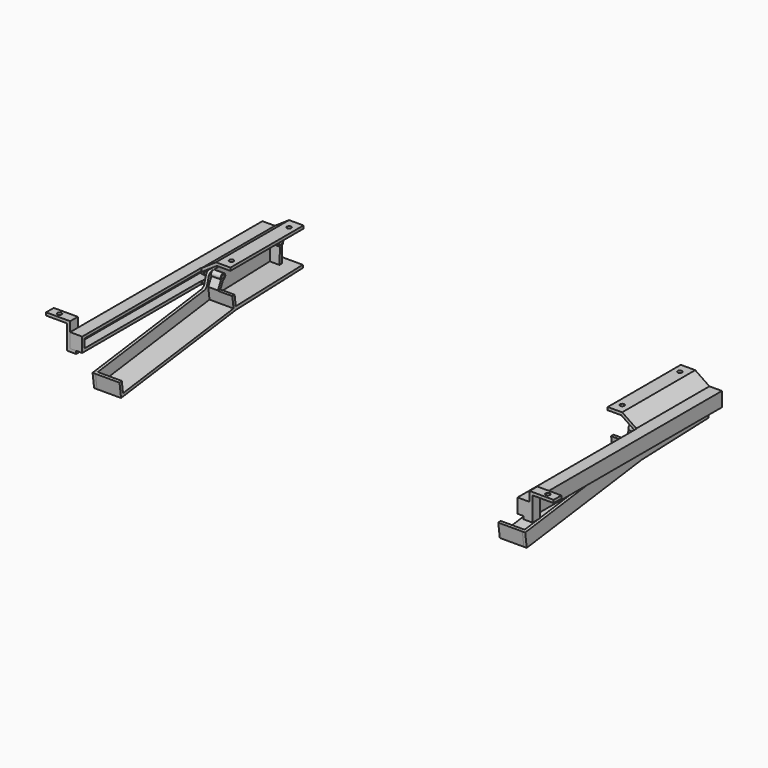
from build123d import *
from build123d import SkipClean  # not in build123d's __all__

# Parameters (mm, degrees)
F0_R      = 4
F0_R_2    = 1.5
F1_DEPTH  = 1.5
F4_DEPTH  = 3
F5_W      = 250
F5_H      = 3
F6_DEPTH  = 10
F8_DEPTH  = 10
F11_DEPTH = 3
F12_R     = 1.75
F13_DEPTH = 3
F15_DEPTH = 25
F19_DEPTH = 10
F24_DEPTH = 3
F27_DEPTH = 250
F28_R     = 2.25
F29_DEPTH = 3
F30_W     = 15.1967487764
F30_H     = 155
F31_DEPTH = 25.001
F36_DEPTH = 3
F37_R     = 5
F40_DEPTH = 10
F41_R     = 2.25
F42_DEPTH = 3


# Not quite as in the source:
# - after a boolean that leaves OpenCascade's solid faulty, fix() repairs it


with BuildPart() as f1:
    # F0 (on Right) → F1 (new body, symmetric)
    with BuildSketch(Plane.YZ):
        Circle(F0_R)
        Circle(F0_R_2, mode=Mode.SUBTRACT)
    extrude(amount=F1_DEPTH, both=True)


with BuildPart() as f1b:
    # F0 (on Right) → F1, piece 2 (new body, symmetric)
    with BuildSketch(Plane.YZ):
        with Locations((75, 0)):
            Circle(F0_R)
        with Locations((75, 0)):
            Circle(F0_R_2, mode=Mode.SUBTRACT)
    extrude(amount=F1_DEPTH, both=True)


with BuildPart() as f4:
    # F3 (on offset) → F4 (new body)
    with BuildSketch(Plane.YZ.offset(-9)):
        Polygon((85, -7.5), (85, 0), (85, 7.5), (-165, 7.5), (-165, -7.5), align=None)
    extrude(amount=F4_DEPTH)

    # F5 (on face) → F6 (join)
    with BuildSketch(Plane.YZ.offset(-6)):
        with Locations((-40, 6)):
            Rectangle(F5_W, F5_H)
    extrude(amount=F6_DEPTH)

    # F7 (on face) → F8 (join)
    with BuildSketch(Plane.YZ.offset(-6)):
        Polygon((-162, 4.5), (-165, 4.5), (-165, -7.5), (85, -7.5), (85, 4.5), (82, 4.5), (82, -4.5), (-162, -4.5), align=None)
    extrude(amount=F8_DEPTH)


with BuildPart() as f11:
    # F10 (on offset) → F11 (new body)
    with BuildSketch(Plane.YZ.offset(5)):
        Polygon((85, -34.7448789892), (85, 3), (-5, 3), (-155, -17), (-151.2994158375, -44.7543812191), align=None)
    extrude(amount=F11_DEPTH)

    # F12 (on face) → F13 (cut, through all)
    with BuildSketch(Plane.YZ.offset(8)):
        Circle(F12_R)
        with Locations((75, 0)):
            Circle(F12_R)
    extrude(amount=-F13_DEPTH, mode=Mode.SUBTRACT)

    # F14 (on face) → F15 (join)
    with BuildSketch(Plane.YZ.offset(8)):
        Polygon((-153.2818716388, -29.8859627089), (-151.2994158375, -44.7543812191), (-1.6240028344, -24.7976594854), (85, -21.7668544501), (85, -18.7668544501), (-2.0859865714, -21.3327814575), (-3.5722099029, -10.1861064713), (-6.5801423378, -10.3257321354), (-4.9941776967, -22.2204669436), (-148.7222232957, -41.3842063568), (-150.3081879368, -29.4894715486), align=None)
    extrude(amount=F15_DEPTH)


with BuildPart() as f17_1:
    # F17: instance of F4
    add(f4.part.mirror(Plane.YZ.offset(230)), clean=False)


with BuildPart() as f17_2:
    # F17: instance of F11
    add(f11.part.mirror(Plane.YZ.offset(230)), clean=False)


with BuildPart() as f17_3:
    # F17: instance of F1
    add(f1.part.mirror(Plane.YZ.offset(230)), clean=False)


with BuildPart() as f17_4:
    # F17: instance of F1b
    add(f1b.part.mirror(Plane.YZ.offset(230)), clean=False)


with BuildPart() as f11_1:
    add(f11.part, clean=False)

    # F18 (on face) → F19 (join)
    with BuildSketch(Plane.YZ.offset(8)):
        with BuildLine():
            Line((0.1918648467, -2.9938583601), (0.9444984824, -1.4732354248))
            ThreePointArc((0.9444984824, -1.4732354248), (-0.7762821201, -1.5684023942), (-1.7441913362, -0.142466076))
            Line((-1.7441913362, -0.142466076), (-2.4968249719, -1.6630890114))
            Line((-2.4968249719, -1.6630890114), (-6.5976568338, -9.9484202638))
            Line((-6.5976568338, -9.9484202638), (-6.5801423378, -10.3257321354))
            Line((-6.5801423378, -10.3257321354), (-3.5722099029, -10.1861064713))
            Line((-3.5722099029, -10.1861064713), (-3.0186622242, -9.4804155204))
            Line((-3.0186622242, -9.4804155204), (0.1918648467, -2.9938583601))
        make_face()
        with BuildLine():
            ThreePointArc((1.75, 0), (1.5354758781, -0.83953191), (0.9444984824, -1.4732354248))
            Line((0.9444984824, -1.4732354248), (0.1918648467, -2.9938583601))
            ThreePointArc((0.1918648467, -2.9938583601), (2.998464197, 0.0959815585), (2.1e-09, 3))
            ThreePointArc((2.1e-09, 3), (-2.6447369462, 1.4161096305), (-2.4968249719, -1.6630890114))
            Line((-2.4968249719, -1.6630890114), (-1.7441913362, -0.142466076))
            ThreePointArc((-1.7441913362, -0.142466076), (-0.0712922215, 1.748547231), (1.75, 0))
        make_face()
        with BuildLine():
            ThreePointArc((76.502361728, -2.7867054701), (78.3375773506, 0.565633976), (75.3913835001, 3))
            ThreePointArc((75.3913835001, 3), (72.4606020485, 0.6407184118), (74.1395130754, -2.7263199445))
            Line((74.1395130754, -2.7263199445), (73.4223152522, -19.1079827435))
            Line((73.4223152522, -19.1079827435), (76.70550069, -19.0112460064))
            Line((76.70550069, -19.0112460064), (76.502361728, -2.7867054701))
        make_face()
        with BuildLine():
            ThreePointArc((75.19569175, 1.7390240766), (76.5575823333, 1.3047912788), (77.1413835001, 0))
            ThreePointArc((77.1413835001, 0), (76.5575823333, -1.3047912788), (75.19569175, -1.7390240766))
            ThreePointArc((75.19569175, -1.7390240766), (73.25, 0), (75.19569175, 1.7390240766))
        make_face(mode=Mode.SUBTRACT)
    with SkipClean():  # cleaning this boolean's faces spoils the solid; the shape is the same uncleaned
        extrude(amount=F19_DEPTH)


with BuildPart() as f21_1:
    # F21: instance of F11
    add(f11_1.part.mirror(Plane.YZ.offset(230)), clean=False)


with BuildPart() as f11_2:
    add(f11_1.part, clean=False)

    # F23 (on face) → F24 (cut, through all)
    with BuildSketch(Plane.YZ.offset(8)):
        Polygon((-1.6240028344, -24.7976594854), (-151.2994158375, -44.7543812191), (85, -34.7448789892), (85, -21.7668544501), align=None)
    extrude(amount=-F24_DEPTH, mode=Mode.SUBTRACT)

    add(f11_2.part.fix(), mode=Mode.REPLACE)


with BuildPart() as f25_1:
    # F25: instance of F11
    add(f11_2.part.mirror(Plane.YZ.offset(230)), clean=False)


with BuildPart() as f4_1:
    add(f4.part, clean=False)

    # F26 (on face) → F27 (join)
    with BuildSketch(Plane.XZ.offset(165)):
        Polygon((18.7617782503, 17.5), (4, 7.5), (4, 4.5), (4.9341931008, 4.5), (5.6825543195, 5.0162506242), (19.6822548463, 14.5), (33.7617782503, 14.5), (33.7617782503, 17.5), align=None)
    extrude(amount=-F27_DEPTH)

    # F28 (on face) → F29 (cut, through all)
    with BuildSketch(Plane.XY.offset(17.5)):
        with Locations((26.7617782503, 75)):
            Circle(F28_R)
        with Locations((26.7617782503, 0)):
            Circle(F28_R)
    extrude(amount=-F29_DEPTH, mode=Mode.SUBTRACT)


with BuildPart() as f31_tool:
    # F30 (on face) → F31 (new body, through all)
    with BuildSketch(Plane.XY.offset(17.5)):
        Polygon((33.7617782503, -10), (26.7617782503, -10), (18.7617782503, -10), (18.7617782503, -165), (33.7617782503, -165), align=None)
        with Locations((11.1634038622, -87.5)):
            Rectangle(F30_W, F30_H)
    extrude(amount=-F31_DEPTH)


with BuildPart() as f4_2:
    add(f4_1.part, clean=False)

    # F31: cut by f31_tool
    add(f31_tool.part, mode=Mode.SUBTRACT)


with BuildPart() as f11_3:
    add(f11_2.part, clean=False)

    # F31: cut by f31_tool
    add(f31_tool.part, mode=Mode.SUBTRACT)

    # F35 (on face) → F36 (cut, through all)
    with BuildSketch(Plane.YZ.offset(8)):
        Polygon((-155, -17), (-153.2818716388, -29.8859627089), (-150.3081879368, -29.4894715486), (-8.9276075771, -10.6387275006), (-5, 3), (-10, 2.3333333333), (-10, -7.501), (-83.7575, -7.501), align=None)
    extrude(amount=-F36_DEPTH, mode=Mode.SUBTRACT)

    # F37
    f37_edges = [f11_3.edges().sort_by_distance(p)[0] for p in [
        (6.5, -8.927608, -10.638728),
        (6.5, -5, 3),
    ]]
    fillet(f37_edges, radius=F37_R)


with BuildPart() as f33_1:
    # F33: instance of F4
    add(f4_2.part.mirror(Plane.YZ.offset(230)), clean=False)

    # F43: F40 across plane


with BuildPart() as f38_1:
    # F38: instance of F11
    add(f11_3.part.mirror(Plane.YZ.offset(230)), clean=False)


with BuildPart() as f40:
    # F39 (on face) → F40 (new body)
    with BuildSketch(Plane.XZ.offset(165)):
        Polygon((-2.717485263, -10.5), (-2.717485263, -7.5), (-9, -7.5), (-9, 7.5), (-9, 17.5), (-34, 17.5), (-34, 14.5), (-12, 14.5), (-12, -10.5), align=None)
    extrude(amount=-F40_DEPTH)

    # F41 (on face) → F42 (cut, through all)
    with BuildSketch(Plane.XY.offset(17.5)):
        with Locations((-24, -160)):
            Circle(F41_R)
    extrude(amount=-F42_DEPTH, mode=Mode.SUBTRACT)


with BuildPart() as f33_1_1:
    add(f33_1.part, clean=False)
    add(f40.part.mirror(Plane.YZ.offset(230)), clean=False)


solid = Compound([f1.part, f1b.part, f17_3.part, f17_4.part, f4_2.part, f11_3.part, f38_1.part, f40.part, f33_1_1.part])
